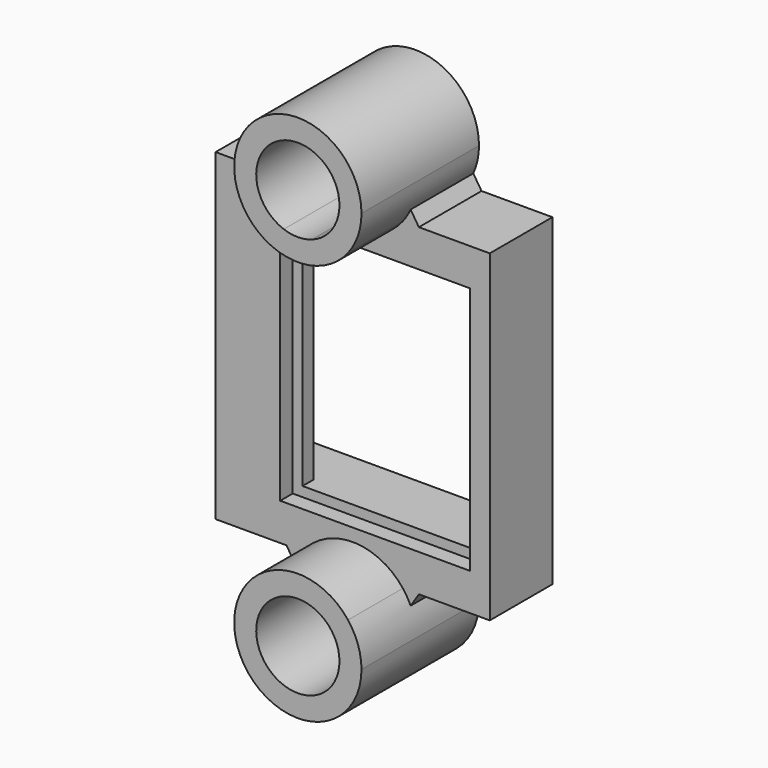
from build123d import *

# Parameters (mm, degrees)
F1_DEPTH    = 8
F3_DEPTH    = 15
F4_T1_DEPTH = 8
F5_W        = 19.4
F5_H        = 25.4
F6_DEPTH    = 1.6
F7_W        = 17.4
F7_H        = 23.4
F8_DEPTH    = 25
F9_W        = 17.6963857411
F9_H        = 23.4
F10_DEPTH   = 5
F11_W       = 1
F11_H       = 16
F12_DEPTH   = 2


# Not quite as in the source:
# - a fillet or chamfer that OpenCascade refuses, or shapes differently, is made with other operations: its cross-section is extruded or revolved along the edge and cut away or added
# - a feature of the source that left no trace in its solid (it failed there, or was rolled back) is left out


with BuildPart() as f1:
    # F0 (on Front) → F1 (new body)
    with BuildSketch(Plane.XZ):
        with BuildLine():
            Line((5.123475383, -16.5), (14, -16.5))
            Line((14, -16.5), (14, 16.5))
            Line((14, 16.5), (5.123475383, 16.5))
            ThreePointArc((5.123475383, 16.5), (0, 14), (-5.123475383, 16.5))
            Line((-5.123475383, 16.5), (-14, 16.5))
            Line((-14, 16.5), (-14, -16.5))
            Line((-14, -16.5), (-5.123475383, -16.5))
            ThreePointArc((-5.123475383, -16.5), (0, -14), (5.123475383, -16.5))
        make_face()
    extrude(amount=F1_DEPTH)

    # F0 (on Front) → F3 (join)
    with BuildSketch(Plane.XZ):
        with BuildLine():
            ThreePointArc((6.5, -20.5), (6.1462423475, -18.3848865266), (5.123475383, -16.5))
            Line((5.123475383, -16.5), (1.4361406616, -16.5))
            ThreePointArc((1.4361406616, -16.5), (3.4760680238, -18.0547083826), (4.25, -20.5))
            ThreePointArc((4.25, -20.5), (-2.4452916174, -23.9760680238), (-1.4361406616, -16.5))
            Line((-1.4361406616, -16.5), (-5.123475383, -16.5))
            ThreePointArc((-5.123475383, -16.5), (-2.1151134734, -26.6462423475), (6.5, -20.5))
        make_face()
        with BuildLine():
            Line((1.4361406616, -16.5), (5.123475383, -16.5))
            ThreePointArc((5.123475383, -16.5), (0, -14), (-5.123475383, -16.5))
            Line((-5.123475383, -16.5), (-1.4361406616, -16.5))
            ThreePointArc((-1.4361406616, -16.5), (0, -16.25), (1.4361406616, -16.5))
        make_face()
        with BuildLine():
            ThreePointArc((-5.123475383, 16.5), (0, 14), (5.123475383, 16.5))
            Line((5.123475383, 16.5), (1.4361406616, 16.5))
            ThreePointArc((1.4361406616, 16.5), (0, 16.25), (-1.4361406616, 16.5))
            Line((-1.4361406616, 16.5), (-5.123475383, 16.5))
        make_face()
        with BuildLine():
            Line((1.4361406616, 16.5), (5.123475383, 16.5))
            ThreePointArc((5.123475383, 16.5), (6.1462423475, 18.3848865266), (6.5, 20.5))
            ThreePointArc((6.5, 20.5), (-2.1151134734, 26.6462423475), (-5.123475383, 16.5))
            Line((-5.123475383, 16.5), (-1.4361406616, 16.5))
            ThreePointArc((-1.4361406616, 16.5), (-2.4452916174, 23.9760680238), (4.25, 20.5))
            ThreePointArc((4.25, 20.5), (3.4760680238, 18.0547083826), (1.4361406616, 16.5))
        make_face()
    extrude(amount=F3_DEPTH)

    # F4: chamfer of 1.9 on 4 edges, made by hand

    # F4_s2 → F4_t1 (join)
    with BuildSketch(Plane.XZ):
        with BuildLine():
            Line((-6.8027454264, 16.4361025598), (-5.876418772, 17.87458352))
            Line((-5.876418772, 17.87458352), (-5.8418237692, 17.8903056629))
            ThreePointArc((-5.8418237692, 17.8903056629), (-5.5354543935, 17.1659051218), (-5.0935227577, 16.5233846154))
            Line((-5.0935227577, 16.5233846154), (-5.123475383, 16.462))
            ThreePointArc((-5.123475383, 16.462), (-5.9631104047, 16.462), (-6.8027454264, 16.3981025598))
            Line((-6.8027454264, 16.3981025598), (-6.8027454264, 16.4361025598))
        make_face()
        with BuildLine():
            Line((5.876418772, 17.87458352), (6.8027454264, 16.4361025598))
            Line((6.8027454264, 16.4361025598), (6.8027454264, 16.3981025598))
            ThreePointArc((6.8027454264, 16.3981025598), (5.9631104047, 16.462), (5.123475383, 16.462))
            Line((5.123475383, 16.462), (5.0935227577, 16.5233846154))
            ThreePointArc((5.0935227577, 16.5233846154), (5.5354543935, 17.1659051218), (5.8418237692, 17.8903056629))
            Line((5.8418237692, 17.8903056629), (5.876418772, 17.87458352))
        make_face()
        with BuildLine():
            Line((6.8027454264, -16.4361025598), (5.876418772, -17.87458352))
            Line((5.876418772, -17.87458352), (5.8418237692, -17.8903056629))
            ThreePointArc((5.8418237692, -17.8903056629), (5.5354543935, -17.1659051218), (5.0935227577, -16.5233846154))
            Line((5.0935227577, -16.5233846154), (5.123475383, -16.462))
            ThreePointArc((5.123475383, -16.462), (5.9631104047, -16.462), (6.8027454264, -16.3981025598))
            Line((6.8027454264, -16.3981025598), (6.8027454264, -16.4361025598))
        make_face()
        with BuildLine():
            Line((-6.8027454264, -16.4361025598), (-5.876418772, -17.87458352))
            Line((-5.876418772, -17.87458352), (-5.8418237692, -17.8903056629))
            ThreePointArc((-5.8418237692, -17.8903056629), (-5.5354543935, -17.1659051218), (-5.0935227577, -16.5233846154))
            Line((-5.0935227577, -16.5233846154), (-5.123475383, -16.462))
            ThreePointArc((-5.123475383, -16.462), (-5.9631104047, -16.462), (-6.8027454264, -16.3981025598))
            Line((-6.8027454264, -16.3981025598), (-6.8027454264, -16.4361025598))
        make_face()
    extrude(amount=F4_T1_DEPTH)

    # F5 (on face) → F6 (cut)
    with BuildSketch(Plane.XZ.offset(8)):
        with Locations((2.3, 0)):
            Rectangle(F5_W, F5_H)
    extrude(amount=-F6_DEPTH, mode=Mode.SUBTRACT)

    # F7 (on face) → F8 (cut)
    with BuildSketch(Plane.XZ.offset(6.4)):
        with Locations((2.3, 0)):
            Rectangle(F7_W, F7_H)
    extrude(amount=-F8_DEPTH, mode=Mode.SUBTRACT)

    # F9 (on face) → F10 (cut)
    with BuildSketch(Plane.XZ):
        with Locations((-5.1518071295, 0)):
            Rectangle(F9_W, F9_H)
    extrude(amount=F10_DEPTH, mode=Mode.SUBTRACT)

    # F11 (on face) → F12 (cut)
    with BuildSketch(Plane.XZ.offset(6.4)):
        with Locations((11.5, 0.4684822634)):
            Rectangle(F11_W, F11_H)
    extrude(amount=-F12_DEPTH, mode=Mode.SUBTRACT)


solid = f1.part
